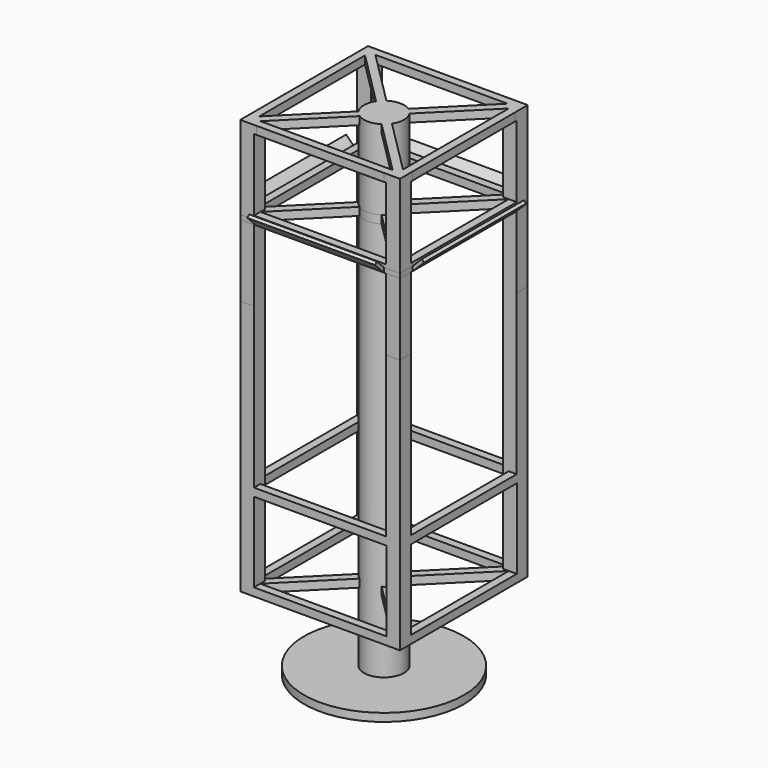
from build123d import *

# Parameters (mm, degrees)
F0_R           = 304.8
F1_DEPTH       = 30.48
F2_R           = 76.2
F3_DEPTH       = 274.32
F4_W           = 609.6
F4_H           = 609.6
F5_DEPTH       = 30.48
F6_R           = 76.2
F6_W           = 52.0326146906
F6_H           = 52.0326146906
F7_DEPTH       = 304.8
F7_DEPTH_BACK  = 30.48
F8_W           = 609.6
F8_H           = 609.6
F8_W_2         = 548.64
F8_H_2         = 548.64
F9_DEPTH       = 30.48
F10_W          = 52.4256
F10_H          = 52.4256
F10_R          = 76.2
F11_DEPTH      = 914.4
F13_DEPTH      = 30.48
F14_W          = 52.4256
F14_H          = 52.4256
F14_R          = 76.2
F15_DEPTH      = 304.8
F15_DEPTH_BACK = 30.48
F16_W          = 609.6
F16_H          = 609.6
F16_W_2        = 548.64
F16_H_2        = 548.64
F17_DEPTH      = 30.48
F20_DEPTH      = 609.6
F22_DEPTH      = 609.6
F23_DEPTH      = 30.48
F24_W          = 60.96
F24_H          = 72.17660923
F24_H_2        = 60.96
F24_H_3        = 74.9131180763
F24_W_2        = 86.0498287201
F24_W_3        = 73.7356283188
F24_H_4        = 73.4948553562
F24_H_5        = 80.3360976696
F24_W_4        = 73.3040608883
F25_DEPTH      = 609.6


# Not quite as in the source:
# - a feature names something its author has since deleted; it is built from what else it names


with BuildPart() as f1:
    # F0 (on Top) → F1 (new body)
    with BuildSketch(Plane.XY):
        Circle(F0_R)
    extrude(amount=F1_DEPTH)

    # F2 (on face) → F3 (join)
    with BuildSketch(Plane.XY.offset(30.48)):
        Circle(F2_R)
    extrude(amount=F3_DEPTH)

    # F4 (on face) → F5 (join)
    with BuildSketch(Plane.XY.offset(304.8)):
        Rectangle(F4_W, F4_H)
        Polygon((-21.5526146906, 0), (-274.32, -252.7673853094), (-274.32, 252.7673853094), align=None, mode=Mode.SUBTRACT)
        Polygon((0, -21.5526146906), (252.7673853094, -274.32), (-252.7673853094, -274.32), align=None, mode=Mode.SUBTRACT)
        Polygon((-252.7673853094, 274.32), (252.7673853094, 274.32), (0, 21.5526146906), align=None, mode=Mode.SUBTRACT)
        Polygon((274.32, 252.7673853094), (274.32, -252.7673853094), (21.5526146906, 0), align=None, mode=Mode.SUBTRACT)
    extrude(amount=F5_DEPTH)

    # F6 (on face) → F7 (join, two sides)
    with BuildSketch(Plane.XY.offset(335.28)) as f7_sk:
        Circle(F6_R)
        with Locations((-278.7836926547, 278.7836926547)):
            Rectangle(F6_W, F6_H)
        with Locations((278.7836926547, 278.7836926547)):
            Rectangle(F6_W, F6_H)
        with Locations((278.7836926547, -278.7836926547)):
            Rectangle(F6_W, F6_H)
        with Locations((-278.7836926547, -278.7836926547)):
            Rectangle(F6_W, F6_H)
    extrude(amount=F7_DEPTH)
    extrude(f7_sk.sketch, amount=-F7_DEPTH_BACK)

    # F8 (on face) → F9 (join)
    with BuildSketch(Plane.XY.offset(640.08)):
        Rectangle(F8_W, F8_H)
        Rectangle(F8_W_2, F8_H_2, mode=Mode.SUBTRACT)
    extrude(amount=F9_DEPTH)

    # F10 (on face) → F11 (join)
    with BuildSketch(Plane.XY.offset(640.08)):
        with Locations((-278.5872, 278.5872)):
            Rectangle(F10_W, F10_H)
        with Locations((-278.5872, -278.5872)):
            Rectangle(F10_W, F10_H)
        with Locations((278.5872, 278.5872)):
            Rectangle(F10_W, F10_H)
        with Locations((278.5872, -278.5872)):
            Rectangle(F10_W, F10_H)
        Circle(F10_R)
    extrude(amount=F11_DEPTH)

    # F12 (on face) → F13 (join)
    with BuildSketch(Plane.XY.offset(1554.48)):
        Polygon((252.3744, -304.8), (304.8, -304.8), (304.8, -252.3744), (304.8, 252.3744), (304.8, 304.8), (252.3744, 304.8), (-252.3744, 304.8), (-304.8, 304.8), (-304.8, 252.3744), (-304.8, -252.3744), (-304.8, -304.8), (-252.3744, -304.8), align=None)
        Polygon((252.3744, -274.32), (-252.3744, -274.32), (0, -21.9456), align=None, mode=Mode.SUBTRACT)
        Polygon((-274.32, -252.3744), (-274.32, 252.3744), (-21.9456, 0), align=None, mode=Mode.SUBTRACT)
        Polygon((21.9456, 0), (274.32, 252.3744), (274.32, -252.3744), align=None, mode=Mode.SUBTRACT)
        Polygon((0, 21.9456), (-252.3744, 274.32), (252.3744, 274.32), align=None, mode=Mode.SUBTRACT)
    extrude(amount=F13_DEPTH)

    # F14 (on face) → F15 (join, two sides)
    with BuildSketch(Plane.XY.offset(1584.96)) as f15_sk:
        with Locations((-278.5872, 278.5872)):
            Rectangle(F14_W, F14_H)
        with Locations((278.5872, 278.5872)):
            Rectangle(F14_W, F14_H)
        with Locations((278.5872, -278.5872)):
            Rectangle(F14_W, F14_H)
        with Locations((-278.5872, -278.5872)):
            Rectangle(F14_W, F14_H)
        Circle(F14_R)
    extrude(amount=F15_DEPTH)
    extrude(f15_sk.sketch, amount=-F15_DEPTH_BACK)

    # F16 (on face) → F17 (join)
    with BuildSketch(Plane.XY.offset(1889.76)):
        Rectangle(F16_W, F16_H)
        Rectangle(F16_W_2, F16_H_2, mode=Mode.SUBTRACT)
    extrude(amount=-F17_DEPTH)

    # F19 (on face) → F20 (join)
    with BuildSketch(Plane.XZ.offset(304.8)):
        Polygon((-347.9052293811, 1597.5852293811), (-304.8, 1554.48), (-274.32, 1554.48), (-274.32, 1571.7220917525), (-304.8, 1571.7220917525), (-339.2841835049, 1606.2062752574), align=None)
        Polygon((274.32, 1554.48), (304.8, 1554.48), (347.9052293811, 1597.5852293811), (339.2841835049, 1606.2062752574), (304.8, 1571.7220917525), (274.32, 1571.7220917525), align=None)
    extrude(amount=-F20_DEPTH)

    # F21 (on face) → F22 (join)
    with BuildSketch(Plane.YZ.offset(304.8)):
        Polygon((274.32, 1571.7220917525), (274.32, 1554.48), (304.8, 1554.48), (347.9052293811, 1597.5852293811), (339.2841835049, 1606.2062752574), (304.8, 1571.7220917525), align=None)
        Polygon((-304.8, 1554.48), (-274.32, 1554.48), (-274.32, 1571.7220917525), (-304.8, 1571.7220917525), (-339.2841835049, 1606.2062752574), (-347.9052293811, 1597.5852293811), align=None)
    extrude(amount=-F22_DEPTH)

    # F18 (on face) → F23 (join)
    with BuildSketch(Plane.XY.offset(1889.76)):
        Polygon((0, 21.9456), (-252.3744, 274.32), (-274.32, 274.32), (-274.32, 252.3744), (-21.9456, 0), (-274.32, -252.3744), (-274.32, -274.32), (-252.3744, -274.32), (0, -21.9456), (252.3744, -274.32), (274.32, -274.32), (274.32, -252.3744), (21.9456, 0), (274.32, 252.3744), (274.32, 274.32), (252.3744, 274.32), align=None)
    extrude(amount=-F23_DEPTH)

    # F24 (on face) → F25 (cut)
    with BuildSketch(Plane.XY.offset(1889.76)):
        with Locations((-274.32, 340.888304615)):
            Rectangle(F24_W, F24_H)
        with Locations((-335.28, 274.32)):
            Rectangle(F24_W, F24_H_2)
        with Locations((274.32, 342.2565590382)):
            Rectangle(F24_W, F24_H_3)
        with Locations((347.82491436, 274.32)):
            Rectangle(F24_W_2, F24_H_2)
        with Locations((341.6678141594, -274.32)):
            Rectangle(F24_W_3, F24_H_2)
        with Locations((274.32, -341.5474276781)):
            Rectangle(F24_W, F24_H_4)
        with Locations((-274.32, -344.9680488348)):
            Rectangle(F24_W, F24_H_5)
        with Locations((-341.4520304441, -274.32)):
            Rectangle(F24_W_4, F24_H_2)
    extrude(amount=-F25_DEPTH, mode=Mode.SUBTRACT)


solid = f1.part
